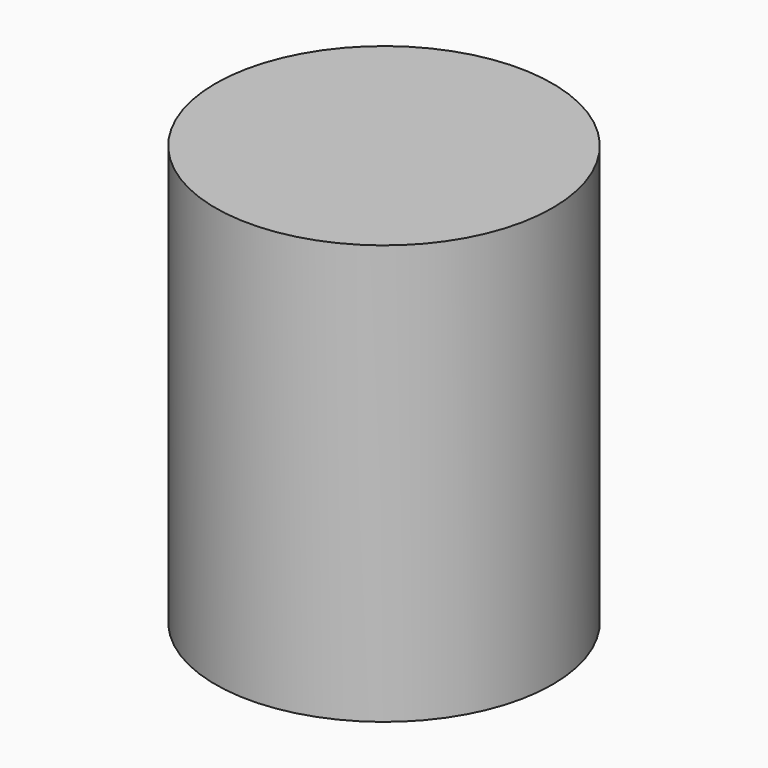
from build123d import *

# Parameters (mm, degrees)
F0_R     = 61.2289564534
F1_DEPTH = 152.4


# Not quite as in the source:
# - the program builds the solid bodies; features that only make, move or delete a surface that nothing else refers to are left out


with BuildPart() as f1:
    # F0 (on Top) → F1 (new body)
    with BuildSketch(Plane.XY):
        Circle(F0_R)
    extrude(amount=F1_DEPTH)


solid = f1.part
